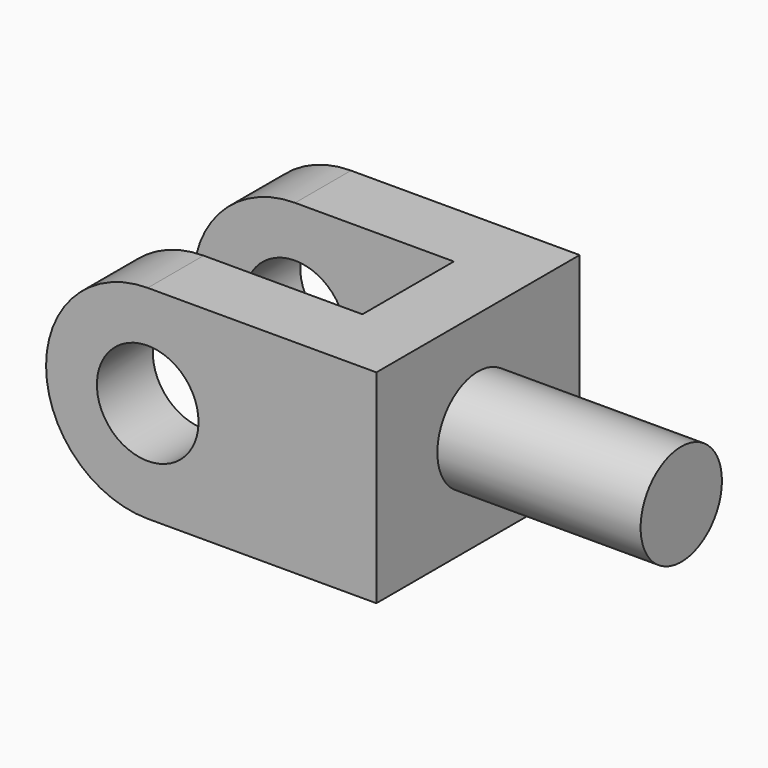
from build123d import *

# Parameters (mm, degrees)
F1_DEPTH = 812.8
F2_R     = 406.39999
F3_R     = 203.2
F4_DEPTH = 1016.001
F5_R     = 203.2
F6_DEPTH = 812.8


# Not quite as in the source:
# - a fillet or chamfer is up to 0.001 mm smaller than in the source, because OpenCascade refuses the exact size


with BuildPart() as f1:
    # F0 (on Top) → F1 (new body)
    with BuildSketch(Plane.XY):
        Polygon((0, 279.4), (0, 0), (1320.8, 0), (1320.8, 1016), (0, 1016), (0, 736.6), (1041.4, 736.6), (1041.4, 279.4), align=None)
    extrude(amount=F1_DEPTH)

    # F2 (radius 406.4 in the source; OpenCascade refuses exactly that, so slightly less here)
    f2_edges = [f1.edges().sort_by_distance(p)[0] for p in [
        (0, 139.7, 812.8),
        (0, 139.7, 0),
        (0, 876.3, 0),
        (0, 876.3, 812.8),
    ]]
    fillet(f2_edges, radius=F2_R)

    # F3 (on face) → F4 (cut, through all)
    with BuildSketch(Plane.XZ):
        with Locations((406.4, 406.4)):
            Circle(F3_R)
    extrude(amount=-F4_DEPTH, mode=Mode.SUBTRACT)

    # F5 (on face) → F6 (join)
    with BuildSketch(Plane.YZ.offset(1320.8)):
        with Locations((508, 406.4)):
            Circle(F5_R)
    extrude(amount=F6_DEPTH)


solid = f1.part
